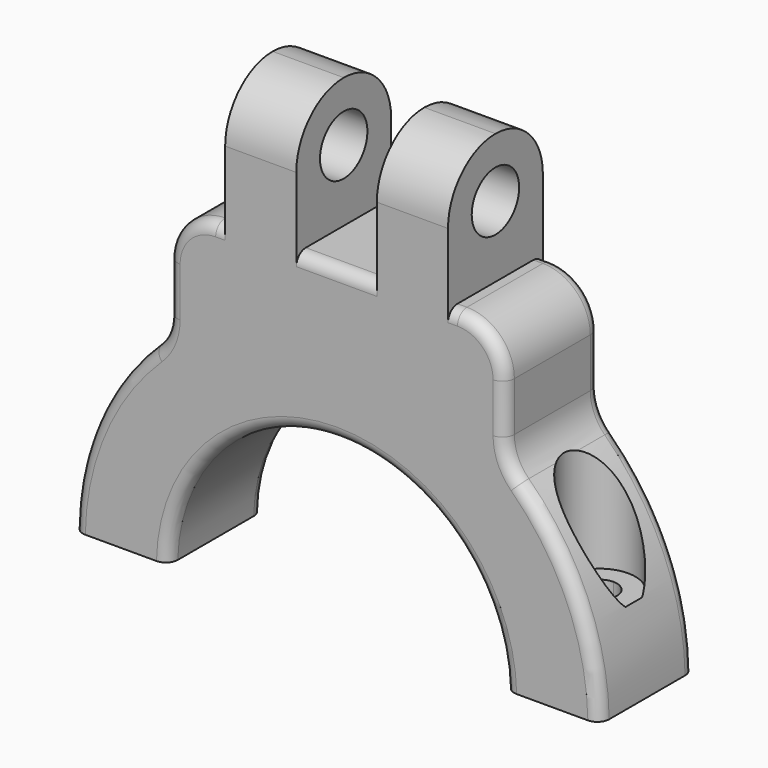
from build123d import *

# Parameters (mm, degrees)
F1_DEPTH  = 12.7
F5_W      = 7.62
F5_H      = 12.7
F6_DEPTH  = 13.97
F8_DEPTH  = 23.876
F9_R      = 6.34999
F10_R     = 5.08
F12_REACH = 53.0526275257
F14_REACH = 53.0526275257
F15_R     = 3.81
F16_DEPTH = 25.4
F17_R     = 1.27


# Not quite as in the source:
# - a fillet or chamfer is up to 0.001 mm smaller than in the source, because OpenCascade refuses the exact size


with BuildPart() as f1:
    # F0 (on Front) → F1 (new body)
    with BuildSketch(Plane.XZ):
        with BuildLine():
            Line((-10.1574255581, 0.381), (0.0040250971, 0.381))
            ThreePointArc((0.0040250971, 0.381), (18.034, 18.034), (36.0639749029, 0.381))
            Line((36.0639749029, 0.381), (46.2254255581, 0.381))
            ThreePointArc((46.2254255581, 0.381), (18.034, 28.194), (-10.1574255581, 0.381))
        make_face()
    extrude(amount=F1_DEPTH)

    # F3 (on offset) → F4 (join, up to the next surface of F1)
    with BuildSketch(Plane.XY.offset(34.29)):
        Polygon((18.034, 0), (0, 0), (0, -12.7), (36.068, -12.7), (36.068, 0), align=None)
    extrude(until=Until.NEXT, dir=(0, 0, -1))

    # F5 (on face) → F6 (join)
    with BuildSketch(Plane.XY.offset(34.29)):
        with Locations((9.906, -6.35)):
            Rectangle(F5_W, F5_H)
        with Locations((26.162, -6.35)):
            Rectangle(F5_W, F5_H)
    extrude(amount=F6_DEPTH)

    # F7 (on face) → F8 (cut, through all)
    with BuildSketch(Plane(origin=(6.096, 0, 0), x_dir=(0, -1, 0), z_dir=(-1, 0, 0))):
        with BuildLine():
            ThreePointArc((6.35, 45.085), (4.1049359697, 39.6649359697), (9.525, 41.91))
            ThreePointArc((9.525, 41.91), (8.5950640303, 44.1550640303), (6.35, 45.085))
        make_face()
    extrude(amount=-F8_DEPTH, mode=Mode.SUBTRACT)

    # F9 (radius 6.35 in the source; OpenCascade refuses exactly that, so slightly less here)
    f9_edges = [f1.edges().sort_by_distance(p)[0] for p in [
        (9.906, -12.7, 48.26),
        (26.162, -12.7, 48.26),
        (9.906, 0, 48.26),
        (26.162, 0, 48.26),
    ]]
    fillet(f9_edges, radius=F9_R)

    # F10
    f10_edges = [f1.edges().sort_by_distance(p)[0] for p in [
        (36.068, -6.35, 34.29),
        (36.068, -6.35, 21.672021),
        (0, -6.35, 34.29),
        (0, -6.35, 21.672021),
    ]]
    fillet(f10_edges, radius=F10_R)

    f12_end = f1.faces().sort_by_distance((-7.8436707665, -6.35, 11.1914159829))[0]
    # F11 (on face) → F12 (cut, up to a face of the model that its end follows)
    with BuildSketch(Plane(origin=(0, 0, 0.381), x_dir=(1, 0, 0), z_dir=(0, 0, -1))):
        with BuildLine():
            ThreePointArc((-3.2479002305, 6.35), (-6.369857112, 7.6431568814), (-5.0767002305, 4.5212))
            ThreePointArc((-5.0767002305, 4.5212), (-3.7835433491, 5.0568431186), (-3.2479002305, 6.35))
        make_face()
    f12_long = extrude(amount=-F12_REACH, mode=Mode.PRIVATE)
    add(split(f12_long, bisect_by=f12_end, keep=Keep.BOTTOM, mode=Mode.PRIVATE), mode=Mode.SUBTRACT)

    f14_end = f1.faces().sort_by_distance((43.9116707665, -6.35, 11.1914159829))[0]
    # F13 (on face) → F14 (cut, up to a face of the model that its end follows)
    with BuildSketch(Plane(origin=(0, 0, 0.381), x_dir=(1, 0, 0), z_dir=(0, 0, -1))):
        with BuildLine():
            ThreePointArc((42.9735002305, 6.35), (39.8515433491, 7.6431568814), (41.1447002305, 4.5212))
            ThreePointArc((41.1447002305, 4.5212), (42.437857112, 5.0568431186), (42.9735002305, 6.35))
        make_face()
    f14_long = extrude(amount=-F14_REACH, mode=Mode.PRIVATE)
    add(split(f14_long, bisect_by=f14_end, keep=Keep.BOTTOM, mode=Mode.PRIVATE), mode=Mode.SUBTRACT)

    # F15 (on face) → F16 (cut)
    with BuildSketch(Plane.XY.offset(34.29)):
        with Locations((-5.0767002305, -6.35)):
            Circle(F15_R)
        with Locations((41.1447002305, -6.35)):
            Circle(F15_R)
    extrude(amount=-F16_DEPTH, mode=Mode.SUBTRACT)

    # F17
    f17_edges = [f1.edges().sort_by_distance(p)[0] for p in [
        (18.034, 0, 18.034),
        (-7.843671, 0, 11.191416),
        (-7.843671, -12.7, 11.191416),
        (43.911671, -12.7, 11.191416),
        (18.034, -12.7, 18.034),
        (43.911671, 0, 11.191416),
        (18.034, -12.7, 34.29),
        (18.034, 0, 34.29),
    ]]
    fillet(f17_edges, radius=F17_R)


solid = f1.part
